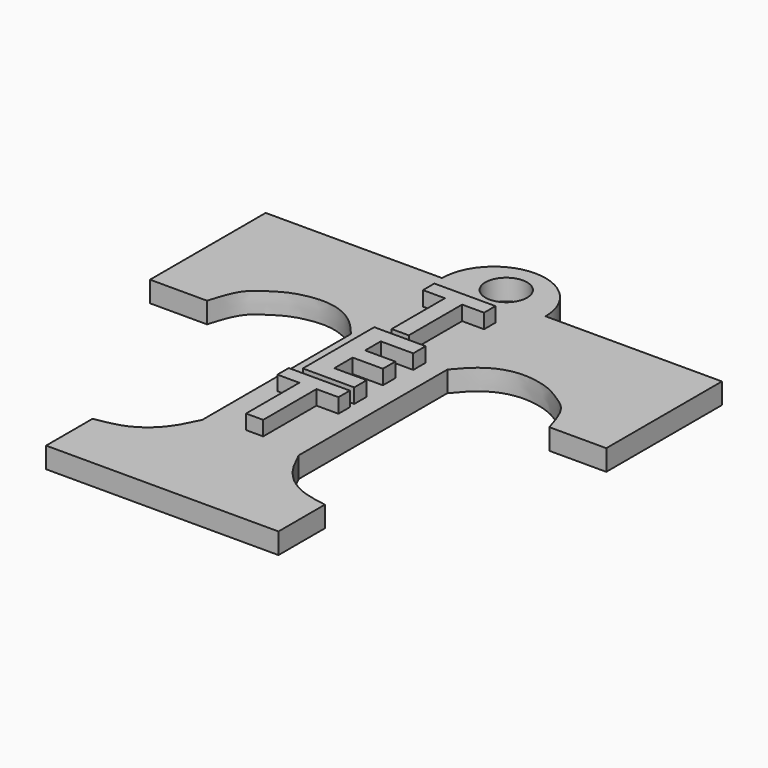
from build123d import *

# Parameters (mm, degrees)
F1_DEPTH       = 2.54
F3_D           = 5.08
F4_TEXT_SIZE   = 13.8163618329
F4_TEXT_SIZE_2 = 15.243052298
F5_DEPTH       = 1.778


# Not quite as in the source:
# - Text() gives the source's letters only with a copy of the font that has no kerning and outlines rounded to 1/6400 em; it was checked with that copy


with BuildPart() as f1:
    # F0 (on Top) → F1 (new body)
    with BuildSketch(Plane.XY):
        with BuildLine():
            Line((22.7953840206, -2.3612247314), (1.2964573689, -2.3612247314))
            Line((1.2964573689, -2.3612247314), (1.2964573689, -19.9816245586))
            Line((1.2964573689, -19.9816245586), (8.2398285158, -19.9816245586))
            add(Edge.make_bspline(
                [(23.2333955355, -16.7752262205), (22.8352937735, -16.2916145801), (21.986652509, -15.2606902456), (20.0344221133, -13.6785598532), (17.4666718071, -12.9970672958), (15.2661637311, -13.2098285143), (13.2328517311, -13.7447034789), (11.4759532907, -14.8608167221), (9.951582089, -15.8844920747), (8.9946472648, -17.515166048), (8.5061138827, -19.1115059901), (8.2398285158, -19.9816245586)],
                knots=[0, 0, 0, 0, 0.105105217, 0.2240548342, 0.3459284125, 0.4576611764, 0.5664371729, 0.6751610054, 0.7761121262, 0.8779652183, 1, 1, 1, 1], degree=3))
            Line((23.2333955355, -16.7752262205), (23.2333955355, -39.4346825778))
            add(Edge.make_bspline(
                [(23.2333955355, -39.4346825778), (22.9230646531, -40.0996081827), (22.3291022631, -41.372252395), (21.2823881414, -42.8785587818), (20.040101999, -44.0774008746), (18.0228111949, -45.2708530432), (16.0226573303, -45.613795239), (14.9399270304, -45.7994379103)],
                knots=[0, 0, 0, 0, 0.198582321, 0.3800795753, 0.5554981457, 0.7593806984, 1, 1, 1, 1], degree=3))
            Line((14.9399270304, -45.7994379103), (14.9399270304, -52.8713911772))
            Line((14.9399270304, -52.8713911772), (43.2661622763, -52.8713911772))
            Line((43.2661622763, -52.8713911772), (43.2661622763, -45.7994379103))
            add(Edge.make_bspline(
                [(34.9726937711, -39.4346825778), (35.2830246535, -40.0996081827), (35.8769870435, -41.372252395), (36.9237011652, -42.8785587818), (38.1659873076, -44.0774008746), (40.1832781117, -45.2708530432), (42.1834319763, -45.613795239), (43.2661622763, -45.7994379103)],
                knots=[0, 0, 0, 0, 0.198582321, 0.3800795753, 0.5554981457, 0.7593806984, 1, 1, 1, 1], degree=3))
            Line((34.9726937711, -39.4346825778), (34.9726937711, -16.7752262205))
            add(Edge.make_bspline(
                [(34.9726937711, -16.7752262205), (35.3707955331, -16.2916145801), (36.2194367976, -15.2606902456), (38.1716671933, -13.6785598532), (40.7394174996, -12.9970672958), (42.9399255756, -13.2098285143), (44.9732375755, -13.7447034789), (46.7301360159, -14.8608167221), (48.2545072176, -15.8844920747), (49.2114420419, -17.515166048), (49.699975424, -19.1115059901), (49.9662607908, -19.9816245586)],
                knots=[0, 0, 0, 0, 0.105105217, 0.2240548342, 0.3459284125, 0.4576611764, 0.5664371729, 0.6751610054, 0.7761121262, 0.8779652183, 1, 1, 1, 1], degree=3))
            Line((49.9662607908, -19.9816245586), (56.9096319377, -19.9816245586))
            Line((56.9096319377, -19.9816245586), (56.9096319377, -2.3612247314))
            Line((56.9096319377, -2.3612247314), (35.410705286, -2.3612247314))
            ThreePointArc((35.410705286, -2.3612247314), (29.1030446533, 3.9464359013), (22.7953840206, -2.3612247314))
        make_face()
    extrude(amount=F1_DEPTH)

    # F3 (through all)
    with Locations(Plane.XY.offset(2.54)):
        with Locations((29.1030446533, -0.4645819135)):
            Hole(F3_D / 2)

    # F4 (on face) → F5 (join)
    with BuildSketch(Plane.XY.offset(2.54)):
        with Locations((24.7871559113, -16.2277920172)):
            Text('T', F4_TEXT_SIZE, font='Open Sans', font_style=FontStyle.BOLD, text_align=(TextAlign.LEFT, TextAlign.BOTTOM))
        with Locations((24.847978726, -27.8515554965)):
            Text('E', F4_TEXT_SIZE_2, font='Open Sans', font_style=FontStyle.BOLD, text_align=(TextAlign.LEFT, TextAlign.BOTTOM))
        with Locations((24.847978726, -38.4877203032)):
            Text('T', F4_TEXT_SIZE, font='Open Sans', font_style=FontStyle.BOLD, text_align=(TextAlign.LEFT, TextAlign.BOTTOM))
    extrude(amount=F5_DEPTH)


solid = f1.part
